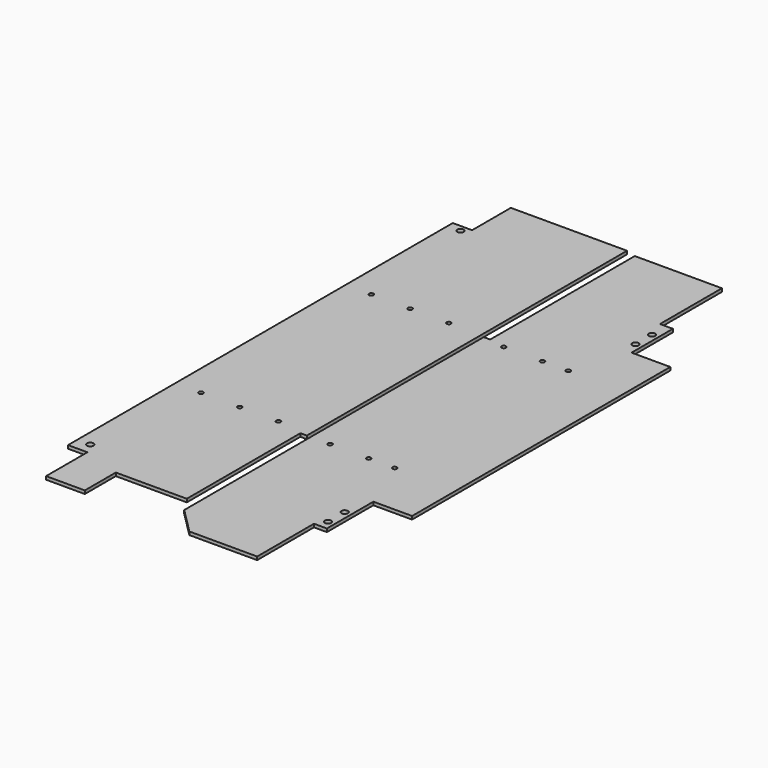
from build123d import *

# Parameters (mm, degrees)
F0_R     = 2.1828125
F0_W     = 19.05
F0_H     = 473.075
F0_R_2   = 3.175
F1_DEPTH = 3.175
F2_R     = 2.1828125
F2_R_2   = 3.175
F2_W     = 38.1
F2_H     = 158.75
F3_DEPTH = 3.175


# Not quite as in the source:
# - a feature names something its author has since deleted; it is built from what else it names


with BuildPart() as f1:
    # F0 (on Top) → F1 (new body)
    with BuildSketch(Plane.XY):
        Polygon((0, 284.1625), (-114.3, 284.1625), (-114.3, 236.5375), (-114.3, -236.5375), (-114.3, -287.3375), (-76.2, -287.3375), (-76.2, -249.2375), (-6.35, -249.2375), (-6.35, -109.5375), (0, -109.5375), align=None)
        with Locations((-107.95, -104.775)):
            Circle(F0_R, mode=Mode.SUBTRACT)
        with Locations((-69.85, -104.775)):
            Circle(F0_R, mode=Mode.SUBTRACT)
        with Locations((-31.75, -104.775)):
            Circle(F0_R, mode=Mode.SUBTRACT)
        with Locations((-107.95, 104.775)):
            Circle(F0_R, mode=Mode.SUBTRACT)
        with Locations((-69.85, 104.775)):
            Circle(F0_R, mode=Mode.SUBTRACT)
        with Locations((-31.75, 104.775)):
            Circle(F0_R, mode=Mode.SUBTRACT)
        with Locations((-123.825, 0)):
            Rectangle(F0_W, F0_H)
        with Locations((-120.65, -225.1075)):
            Circle(F0_R_2, mode=Mode.SUBTRACT)
        with Locations((-120.65, 230.1875)):
            Circle(F0_R_2, mode=Mode.SUBTRACT)
    extrude(amount=F1_DEPTH)


with BuildPart() as f3:
    # F2 (on face) → F3 (new body)
    with BuildSketch(Plane(origin=(0, 0, 0), x_dir=(1, 0, 0), z_dir=(0, 0, -1))):
        Polygon((6.35, -107.95), (6.35, -285.75), (92.075, -285.75), (92.075, -209.55), (92.075, 0), (92.075, 215.9), (92.075, 285.75), (25.4, 285.75), (0, 260.35), (0, 109.5375), (0, -107.95), align=None)
        with Locations((22.225, -104.775)):
            Circle(F2_R, mode=Mode.SUBTRACT)
        with Locations((60.325, -104.775)):
            Circle(F2_R, mode=Mode.SUBTRACT)
        with Locations((85.725, -104.775)):
            Circle(F2_R, mode=Mode.SUBTRACT)
        with Locations((19.05, 104.775)):
            Circle(F2_R, mode=Mode.SUBTRACT)
        with Locations((57.15, 104.775)):
            Circle(F2_R, mode=Mode.SUBTRACT)
        with Locations((82.55, 104.775)):
            Circle(F2_R, mode=Mode.SUBTRACT)
        Polygon((92.075, 0), (92.075, -209.55), (104.775, -209.55), (104.775, -158.75), (104.775, 0), align=None)
        with Locations((98.425, -191.77)):
            Circle(F2_R_2, mode=Mode.SUBTRACT)
        with Locations((98.425, -171.45)):
            Circle(F2_R_2, mode=Mode.SUBTRACT)
        Polygon((92.075, 215.9), (92.075, 0), (104.775, 0), (104.775, 158.75), (104.775, 215.9), align=None)
        with Locations((98.425, 186.055)):
            Circle(F2_R_2, mode=Mode.SUBTRACT)
        with Locations((98.425, 206.629)):
            Circle(F2_R_2, mode=Mode.SUBTRACT)
        with Locations((123.825, -79.375)):
            Rectangle(F2_W, F2_H)
        with Locations((123.825, 79.375)):
            Rectangle(F2_W, F2_H)
    extrude(amount=F3_DEPTH)


solid = Compound([f1.part, f3.part])
